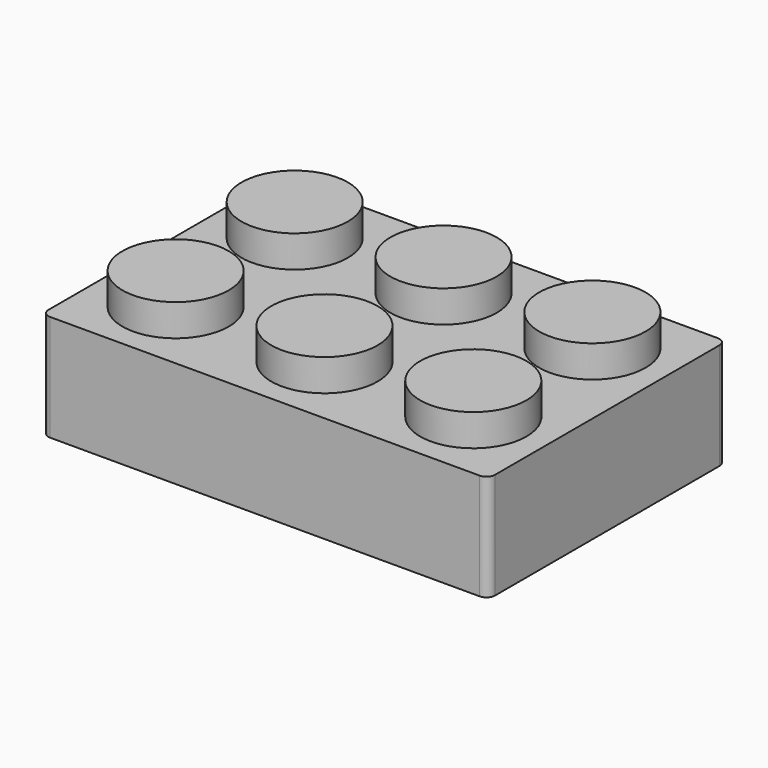
from build123d import *

# Parameters (mm, degrees)
F0_W     = 105
F0_H     = 70
F1_DEPTH = 25
F2_R     = 12.5
F3_DEPTH = 7.5
F4_T     = -5
F6_W     = 95
F6_H     = 2.5
F7_DEPTH = 14.9
F8_W     = 2.5
F8_H     = 60
F9_DEPTH = 19.9
F10_R    = 5
F11_R    = 2


# Not quite as in the source:
# - an extrude ends at something that could not be found from the text; its depth is read off the source's solid


with BuildPart() as f1:
    # F0 (on Top) → F1 (new body)
    with BuildSketch(Plane.XY):
        with Locations((52.5, -35)):
            Rectangle(F0_W, F0_H)
    extrude(amount=F1_DEPTH)

    # F2 (on face) → F3 (join)
    with BuildSketch(Plane.XY.offset(25)):
        with Locations((17.5, -17.5)):
            Circle(F2_R)
        with Locations((52.5, -17.5)):
            Circle(F2_R)
        with Locations((87.5, -17.5)):
            Circle(F2_R)
        with Locations((17.5, -52.5)):
            Circle(F2_R)
        with Locations((52.5, -52.5)):
            Circle(F2_R)
        with Locations((87.5, -52.5)):
            Circle(F2_R)
    extrude(amount=F3_DEPTH)

    # F4
    f4_openings = [f1.faces().sort_by_distance(p)[0] for p in [
        (52.5, -35, 0),
    ]]
    offset(amount=F4_T, openings=f4_openings, kind=Kind.INTERSECTION)

    # F6 (on offset) → F7 (join, through all)
    with BuildSketch(Plane.XY.offset(5.1)):
        with Locations((52.5, -35)):
            Rectangle(F6_W, F6_H)
    extrude(amount=F7_DEPTH)

    # F8 (on offset) → F9 (join, through all)
    with BuildSketch(Plane.XY.offset(5.1)):
        with Locations((36.25, -35)):
            Rectangle(F8_W, F8_H)
        with Locations((68.75, -35)):
            Rectangle(F8_W, F8_H)
    extrude(amount=F9_DEPTH)

    # F10
    f10_edges = [f1.edges().sort_by_distance(p)[0] for p in [
        (5, -65, 10),
        (5, -5, 10),
        (100, -65, 10),
        (100, -5, 10),
    ]]
    fillet(f10_edges, radius=F10_R)

    # F11
    f11_edges = [f1.edges().sort_by_distance(p)[0] for p in [
        (105, -70, 12.5),
        (0, -70, 12.5),
        (0, 0, 12.5),
        (105, 0, 12.5),
    ]]
    fillet(f11_edges, radius=F11_R)


solid = f1.part
